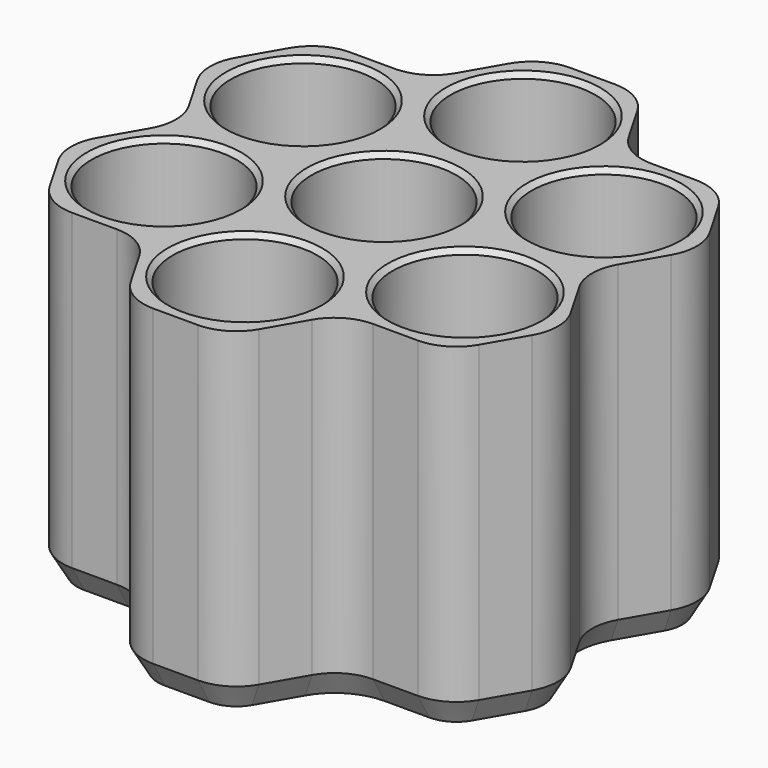
from build123d import *

# Parameters (mm, degrees)
F0_R         = 7.5
F1_DEPTH     = 35
F2_DEPTH     = 2
F3_SIZE      = 0.5
F4_R         = 5
F5_T1_DEPTH  = 4.6188021535
F5_T3_DEPTH  = 4.6188021535
F5_T5_DEPTH  = 4.6188021535
F5_T7_DEPTH  = 4.6188021535
F5_T9_DEPTH  = 4.6188021535
F5_T11_DEPTH = 4.6188021535
F5_T13_DEPTH = 4.6188021535
F5_T15_DEPTH = 4.6188021535
F5_T17_DEPTH = 4.6188021535
F5_T19_DEPTH = 4.6188021535
F5_T21_DEPTH = 4.6188021535
F5_T23_DEPTH = 4.6188021535
F5_T25_DEPTH = 4.6188021535
F5_T27_DEPTH = 4.6188021535
F5_T29_DEPTH = 4.6188021535
F5_T32_ANGLE = 60
F5_T34_ANGLE = 60
F5_T36_ANGLE = 60
F5_T38_ANGLE = 60
F5_T40_ANGLE = 60
F5_T42_ANGLE = 60
F5_T44_ANGLE = 60
F5_T46_ANGLE = 60
F5_T48_ANGLE = 60
F5_T50_ANGLE = 60
F5_T52_ANGLE = 60
F5_T54_ANGLE = 60
F5_T56_ANGLE = 60
F5_T58_ANGLE = 60
F5_T60_ANGLE = 60
F5_T62_ANGLE = 60
F5_T64_ANGLE = 60
F5_T66_ANGLE = 60


# Not quite as in the source:
# - a fillet or chamfer that OpenCascade refuses, or shapes differently, is made with other operations: its cross-section is extruded or revolved along the edge and cut away or added


with BuildPart() as f1:
    # F0 (on Top) → F1 (new body)
    with BuildSketch(Plane.XY):
        Polygon((-10.3923048454, 18), (-5.1961524227, 9), (5.1961524227, 9), (10.3923048454, 18), (5.1961524227, 27), (-5.1961524227, 27), align=None)
        with Locations((0, 18)):
            Circle(F0_R, mode=Mode.SUBTRACT)
        Polygon((5.1961524227, 9), (-5.1961524227, 9), (-10.3923048454, 0), (-5.1961524227, -9), (5.1961524227, -9), (10.3923048454, 0), align=None)
        Circle(F0_R, mode=Mode.SUBTRACT)
        Polygon((-10.3923048454, 0), (-5.1961524227, 9), (-10.3923048454, 18), (-20.7846096908, 18), (-25.9807621135, 9), (-20.7846096908, 0), align=None)
        with Locations((-15.5884572681, 9)):
            Circle(F0_R, mode=Mode.SUBTRACT)
        Polygon((10.3923048454, 18), (5.1961524227, 9), (10.3923048454, 0), (20.7846096908, 0), (25.9807621135, 9), (20.7846096908, 18), align=None)
        with Locations((15.5884572681, 9)):
            Circle(F0_R, mode=Mode.SUBTRACT)
        Polygon((-5.1961524227, -9), (-10.3923048454, 0), (-20.7846096908, 0), (-25.9807621135, -9), (-20.7846096908, -18), (-10.3923048454, -18), align=None)
        with Locations((-15.5884572681, -9)):
            Circle(F0_R, mode=Mode.SUBTRACT)
        Polygon((20.7846096908, 0), (10.3923048454, 0), (5.1961524227, -9), (10.3923048454, -18), (20.7846096908, -18), (25.9807621135, -9), align=None)
        with Locations((15.5884572681, -9)):
            Circle(F0_R, mode=Mode.SUBTRACT)
        Polygon((5.1961524227, -9), (-5.1961524227, -9), (-10.3923048454, -18), (-5.1961524227, -27), (5.1961524227, -27), (10.3923048454, -18), align=None)
        with Locations((0, -18)):
            Circle(F0_R, mode=Mode.SUBTRACT)
    extrude(amount=F1_DEPTH)

    # F0 (on Top) → F2 (join)
    with BuildSketch(Plane.XY):
        with Locations((-15.5884572681, 9)):
            Circle(F0_R)
        with Locations((-15.5884572681, -9)):
            Circle(F0_R)
        with Locations((0, 18)):
            Circle(F0_R)
        Circle(F0_R)
        with Locations((15.5884572681, 9)):
            Circle(F0_R)
        with Locations((15.5884572681, -9)):
            Circle(F0_R)
        with Locations((0, -18)):
            Circle(F0_R)
    extrude(amount=F2_DEPTH)

    # F3
    f3_edges = [f1.edges().sort_by_distance(p)[0] for p in [
        (-7.5, 18, 35),
        (-23.088457, 9, 35),
        (-7.5, 0, 35),
        (-23.088457, -9, 35),
        (8.088457, 9, 35),
        (8.088457, -9, 35),
        (-7.5, -18, 35),
    ]]
    chamfer(f3_edges, length=F3_SIZE)

    # F4
    f4_edges = [f1.edges().sort_by_distance(p)[0] for p in [
        (-25.980762, 9, 17.5),
        (-20.78461, 18, 17.5),
        (-10.392305, 18, 17.5),
        (-5.196152, 27, 17.5),
        (5.196152, 27, 17.5),
        (10.392305, 18, 17.5),
        (20.78461, 18, 17.5),
        (25.980762, 9, 17.5),
        (20.78461, 0, 17.5),
        (25.980762, -9, 17.5),
        (20.78461, -18, 17.5),
        (10.392305, -18, 17.5),
        (5.196152, -27, 17.5),
        (-5.196152, -27, 17.5),
        (-10.392305, -18, 17.5),
        (-20.78461, -18, 17.5),
        (-25.980762, -9, 17.5),
        (-20.78461, 0, 17.5),
    ]]
    fillet(f4_edges, radius=F4_R)

    # F5: chamfer of 1.5 x 2.5980762114 on 36 edges, made by hand

    # F5_s2 → F5_t1 (cut)
    with BuildSketch(Plane.YZ.offset(13.2790561914)):
        Polygon((-18, 2.5980762114), (-16.5, 0), (-18, 0), align=None)
        Polygon((18, 2.5980762114), (16.5, 0), (18, 0), align=None)
    extrude(amount=F5_T1_DEPTH, mode=Mode.SUBTRACT)

    # F5_s4 → F5_t3 (cut)
    with BuildSketch(Plane(origin=(-8.9489291724, -15.5, 0), x_dir=(0, 0, 1), z_dir=(0.5, 0.8660254038, 0))):
        Polygon((2.5980762114, 18), (0, 16.5), (0, 18), align=None)
    extrude(amount=F5_T3_DEPTH, mode=Mode.SUBTRACT)

    # F5_s6 → F5_t5 (cut)
    with BuildSketch(Plane(origin=(-1.1547005384, -2, 0), x_dir=(0, 0, 1), z_dir=(0.5, 0.8660254038, 0))):
        Polygon((2.5980762114, 27), (0, 25.5), (0, 27), align=None)
    extrude(amount=F5_T5_DEPTH, mode=Mode.SUBTRACT)

    # F5_s8 → F5_t7 (cut)
    with BuildSketch(Plane.YZ.offset(-2.3094010768)):
        Polygon((-27, 2.5980762114), (-25.5, 0), (-27, 0), align=None)
        Polygon((27, 2.5980762114), (25.5, 0), (27, 0), align=None)
    extrude(amount=F5_T7_DEPTH, mode=Mode.SUBTRACT)

    # F5_s10 → F5_t9 (cut)
    with BuildSketch(Plane(origin=(8.9489291724, -15.5, 0), x_dir=(0, 0, 1), z_dir=(-0.5, 0.8660254038, 0))):
        Polygon((2.5980762114, 18), (0, 16.5), (0, 18), align=None)
    extrude(amount=F5_T9_DEPTH, mode=Mode.SUBTRACT)

    # F5_s12 → F5_t11 (cut)
    with BuildSketch(Plane(origin=(6.6395280957, -11.5, 0), x_dir=(0, 0, 1), z_dir=(0.5, -0.8660254038, 0))):
        Polygon((2.5980762114, 18), (0, 16.5), (0, 18), align=None)
    extrude(amount=F5_T11_DEPTH, mode=Mode.SUBTRACT)

    # F5_s14 → F5_t13 (cut)
    with BuildSketch(Plane(origin=(6.6395280957, 11.5, 0), x_dir=(0, 0, 1), z_dir=(0.5, 0.8660254038, 0))):
        Polygon((2.5980762114, 18), (0, 16.5), (0, 18), align=None)
    extrude(amount=F5_T13_DEPTH, mode=Mode.SUBTRACT)

    # F5_s16 → F5_t15 (cut)
    with BuildSketch(Plane.YZ.offset(-17.8978583449)):
        Polygon((-18, 2.5980762114), (-16.5, 0), (-18, 0), align=None)
        Polygon((18, 2.5980762114), (16.5, 0), (18, 0), align=None)
    extrude(amount=F5_T15_DEPTH, mode=Mode.SUBTRACT)

    # F5_s18 → F5_t17 (cut)
    with BuildSketch(Plane(origin=(1.1547005384, -2, 0), x_dir=(0, 0, 1), z_dir=(-0.5, 0.8660254038, 0))):
        Polygon((2.5980762114, 27), (0, 25.5), (0, 27), align=None)
    extrude(amount=F5_T17_DEPTH, mode=Mode.SUBTRACT)

    # F5_s20 → F5_t19 (cut)
    with BuildSketch(Plane(origin=(-1.1547005384, 2, 0), x_dir=(0, 0, 1), z_dir=(0.5, -0.8660254038, 0))):
        Polygon((2.5980762114, 27), (0, 25.5), (0, 27), align=None)
    extrude(amount=F5_T19_DEPTH, mode=Mode.SUBTRACT)

    # F5_s22 → F5_t21 (cut)
    with BuildSketch(Plane(origin=(-6.6395280957, -11.5, 0), x_dir=(0, 0, 1), z_dir=(-0.5, -0.8660254038, 0))):
        Polygon((2.5980762114, 18), (0, 16.5), (0, 18), align=None)
    extrude(amount=F5_T21_DEPTH, mode=Mode.SUBTRACT)

    # F5_s24 → F5_t23 (cut)
    with BuildSketch(Plane(origin=(-6.6395280957, 11.5, 0), x_dir=(0, 0, 1), z_dir=(-0.5, 0.8660254038, 0))):
        Polygon((2.5980762114, 18), (0, 16.5), (0, 18), align=None)
    extrude(amount=F5_T23_DEPTH, mode=Mode.SUBTRACT)

    # F5_s26 → F5_t25 (cut)
    with BuildSketch(Plane(origin=(-8.9489291724, 15.5, 0), x_dir=(0, 0, 1), z_dir=(0.5, -0.8660254038, 0))):
        Polygon((2.5980762114, 18), (0, 16.5), (0, 18), align=None)
    extrude(amount=F5_T25_DEPTH, mode=Mode.SUBTRACT)

    # F5_s28 → F5_t27 (cut)
    with BuildSketch(Plane(origin=(1.1547005384, 2, 0), x_dir=(0, 0, 1), z_dir=(-0.5, -0.8660254038, 0))):
        Polygon((2.5980762114, 27), (0, 25.5), (0, 27), align=None)
    extrude(amount=F5_T27_DEPTH, mode=Mode.SUBTRACT)

    # F5_s30 → F5_t29 (cut)
    with BuildSketch(Plane(origin=(8.9489291724, 15.5, 0), x_dir=(0, 0, 1), z_dir=(-0.5, -0.8660254038, 0))):
        Polygon((2.5980762114, 18), (0, 16.5), (0, 18), align=None)
    extrude(amount=F5_T29_DEPTH, mode=Mode.SUBTRACT)

    # F5_s31 → F5_t32 (revolve, cut)
    with BuildSketch(Plane.YZ.offset(13.2790561914)):
        Polygon((-18, 2.5980762114), (-16.5, 0), (-18, 0), align=None)
    revolve(axis=Axis((13.2790561914, -23, 0), (0, 0, 1)), revolution_arc=F5_T32_ANGLE, mode=Mode.SUBTRACT)

    # F5_s33 → F5_t34 (revolve, cut)
    with BuildSketch(Plane.YZ.offset(17.8978583449)):
        Polygon((-18, 2.5980762114), (-16.5, 0), (-18, 0), align=None)
    revolve(axis=Axis((17.8978583449, -13, 0), (0, 0, 1)), revolution_arc=F5_T34_ANGLE, mode=Mode.SUBTRACT)

    # F5_s35 → F5_t36 (revolve, cut)
    with BuildSketch(Plane.YZ.offset(2.3094010768)):
        Polygon((-27, 2.5980762114), (-25.5, 0), (-27, 0), align=None)
    revolve(axis=Axis((2.3094010768, -22, 0), (0, 0, 1)), revolution_arc=F5_T36_ANGLE, mode=Mode.SUBTRACT)

    # F5_s37 → F5_t38 (revolve, cut)
    with BuildSketch(Plane(origin=(1.1547005384, 2, 0), x_dir=(0, 0, 1), z_dir=(-0.5, -0.8660254038, 0))):
        Polygon((2.5980762114, -27), (0, -25.5), (0, -27), align=None)
    revolve(axis=Axis((20.2072594216, -9, 0), (0, 0, 1)), revolution_arc=F5_T38_ANGLE, mode=Mode.SUBTRACT)

    # F5_s39 → F5_t40 (revolve, cut)
    with BuildSketch(Plane(origin=(8.9489291724, -15.5, 0), x_dir=(0, 0, 1), z_dir=(-0.5, 0.8660254038, 0))):
        Polygon((2.5980762114, -18), (0, -16.5), (0, -18), align=None)
    revolve(axis=Axis((-2.3094010768, -22, 0), (0, 0, 1)), revolution_arc=F5_T40_ANGLE, mode=Mode.SUBTRACT)

    # F5_s41 → F5_t42 (revolve, cut)
    with BuildSketch(Plane(origin=(6.6395280957, -11.5, 0), x_dir=(0, 0, 1), z_dir=(0.5, -0.8660254038, 0))):
        Polygon((2.5980762114, -18), (0, -16.5), (0, -18), align=None)
    revolve(axis=Axis((26.5581123827, 0, 0), (0, 0, -1)), revolution_arc=F5_T42_ANGLE, mode=Mode.SUBTRACT)

    # F5_s43 → F5_t44 (revolve, cut)
    with BuildSketch(Plane.YZ.offset(-13.2790561914)):
        Polygon((-18, 2.5980762114), (-16.5, 0), (-18, 0), align=None)
    revolve(axis=Axis((-13.2790561914, -23, 0), (0, 0, -1)), revolution_arc=F5_T44_ANGLE, mode=Mode.SUBTRACT)

    # F5_s45 → F5_t46 (revolve, cut)
    with BuildSketch(Plane(origin=(8.9489291724, 15.5, 0), x_dir=(0, 0, 1), z_dir=(-0.5, -0.8660254038, 0))):
        Polygon((2.5980762114, -18), (0, -16.5), (0, -18), align=None)
    revolve(axis=Axis((20.2072594216, 9, 0), (0, 0, 1)), revolution_arc=F5_T46_ANGLE, mode=Mode.SUBTRACT)

    # F5_s47 → F5_t48 (revolve, cut)
    with BuildSketch(Plane(origin=(1.1547005384, -2, 0), x_dir=(0, 0, 1), z_dir=(-0.5, 0.8660254038, 0))):
        Polygon((2.5980762114, -27), (0, -25.5), (0, -27), align=None)
    revolve(axis=Axis((-17.8978583449, -13, 0), (0, 0, 1)), revolution_arc=F5_T48_ANGLE, mode=Mode.SUBTRACT)

    # F5_s49 → F5_t50 (revolve, cut)
    with BuildSketch(Plane(origin=(-1.1547005384, 2, 0), x_dir=(0, 0, 1), z_dir=(0.5, -0.8660254038, 0))):
        Polygon((2.5980762114, -27), (0, -25.5), (0, -27), align=None)
    revolve(axis=Axis((17.8978583449, 13, 0), (0, 0, 1)), revolution_arc=F5_T50_ANGLE, mode=Mode.SUBTRACT)

    # F5_s51 → F5_t52 (revolve, cut)
    with BuildSketch(Plane(origin=(-8.9489291724, -15.5, 0), x_dir=(0, 0, 1), z_dir=(0.5, 0.8660254038, 0))):
        Polygon((2.5980762114, -18), (0, -16.5), (0, -18), align=None)
    revolve(axis=Axis((-20.2072594216, -9, 0), (0, 0, 1)), revolution_arc=F5_T52_ANGLE, mode=Mode.SUBTRACT)

    # F5_s53 → F5_t54 (revolve, cut)
    with BuildSketch(Plane.YZ.offset(13.2790561914)):
        Polygon((18, 2.5980762114), (16.5, 0), (18, 0), align=None)
    revolve(axis=Axis((13.2790561914, 23, 0), (0, 0, -1)), revolution_arc=F5_T54_ANGLE, mode=Mode.SUBTRACT)

    # F5_s55 → F5_t56 (revolve, cut)
    with BuildSketch(Plane(origin=(-6.6395280957, 11.5, 0), x_dir=(0, 0, 1), z_dir=(-0.5, 0.8660254038, 0))):
        Polygon((2.5980762114, -18), (0, -16.5), (0, -18), align=None)
    revolve(axis=Axis((-26.5581123827, 0, 0), (0, 0, -1)), revolution_arc=F5_T56_ANGLE, mode=Mode.SUBTRACT)

    # F5_s57 → F5_t58 (revolve, cut)
    with BuildSketch(Plane(origin=(-8.9489291724, 15.5, 0), x_dir=(0, 0, 1), z_dir=(0.5, -0.8660254038, 0))):
        Polygon((2.5980762114, -18), (0, -16.5), (0, -18), align=None)
    revolve(axis=Axis((2.3094010768, 22, 0), (0, 0, 1)), revolution_arc=F5_T58_ANGLE, mode=Mode.SUBTRACT)

    # F5_s59 → F5_t60 (revolve, cut)
    with BuildSketch(Plane(origin=(-1.1547005384, -2, 0), x_dir=(0, 0, 1), z_dir=(0.5, 0.8660254038, 0))):
        Polygon((2.5980762114, -27), (0, -25.5), (0, -27), align=None)
    revolve(axis=Axis((-20.2072594216, 9, 0), (0, 0, 1)), revolution_arc=F5_T60_ANGLE, mode=Mode.SUBTRACT)

    # F5_s61 → F5_t62 (revolve, cut)
    with BuildSketch(Plane.YZ.offset(-2.3094010768)):
        Polygon((27, 2.5980762114), (25.5, 0), (27, 0), align=None)
    revolve(axis=Axis((-2.3094010768, 22, 0), (0, 0, 1)), revolution_arc=F5_T62_ANGLE, mode=Mode.SUBTRACT)

    # F5_s63 → F5_t64 (revolve, cut)
    with BuildSketch(Plane.YZ.offset(-17.8978583449)):
        Polygon((18, 2.5980762114), (16.5, 0), (18, 0), align=None)
    revolve(axis=Axis((-17.8978583449, 13, 0), (0, 0, 1)), revolution_arc=F5_T64_ANGLE, mode=Mode.SUBTRACT)

    # F5_s65 → F5_t66 (revolve, cut)
    with BuildSketch(Plane(origin=(6.6395280957, 11.5, 0), x_dir=(0, 0, 1), z_dir=(0.5, 0.8660254038, 0))):
        Polygon((2.5980762114, -18), (0, -16.5), (0, -18), align=None)
    revolve(axis=Axis((-13.2790561914, 23, 0), (0, 0, -1)), revolution_arc=F5_T66_ANGLE, mode=Mode.SUBTRACT)


solid = f1.part
